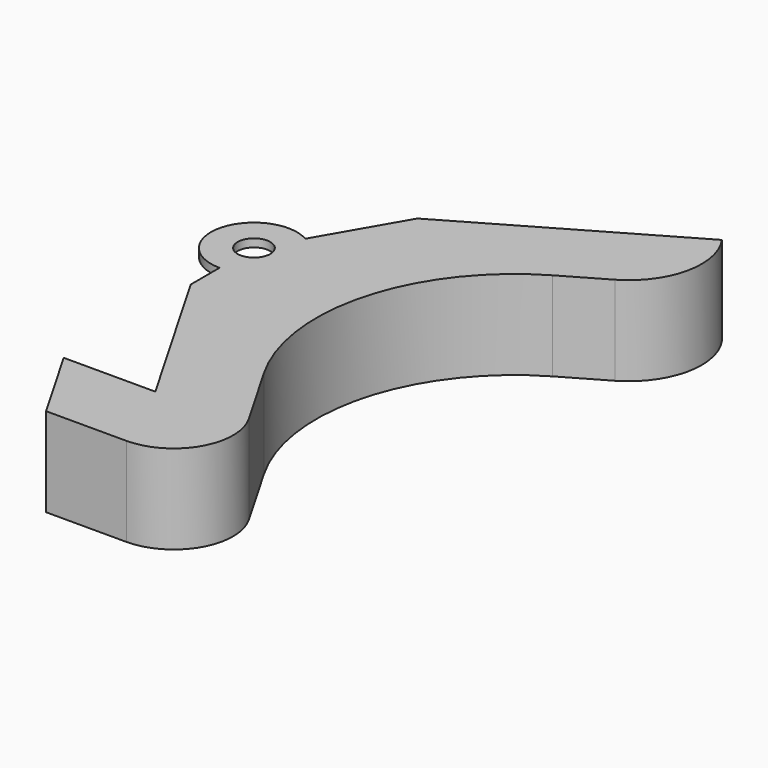
from build123d import *

# Parameters (mm, degrees)
F1_DEPTH    = 9
F2_T        = -1.625
F3_R        = 4.65
F4_DEPTH    = 5.75
F6_DEPTH    = 9
F7_T4_DEPTH = 11.5292765407
F8_R        = 1.5
F9_R        = 1.5
F11_DEPTH   = 25
F12_R       = 1.65
F13_DEPTH   = 0.8125
F14_R       = 4.65
F14_R_2     = 1.65
F15_DEPTH   = 0.8125
F17_DEPTH   = 25
F19_DEPTH   = 25


# Not quite as in the source:
# - a fillet or chamfer that OpenCascade refuses, or shapes differently, is made with other operations: its cross-section is extruded or revolved along the edge and cut away or added


with BuildPart() as f1:
    # F0 (on Top) → F1 (new body)
    with BuildSketch(Plane.XY):
        with BuildLine():
            Line((-2.2380131875, 10.0346875), (0, 9.35))
            Line((0, 9.35), (9.2696152423, -6.7054445662))
            Line((9.2696152423, -6.7054445662), (0, -6.7054445662))
            Line((0, -6.7054445662), (4.6188021535, -14.7054445662))
            Line((4.6188021535, -14.7054445662), (12.7337168574, -14.7054445662))
            ThreePointArc((12.7337168574, -14.7054445662), (17.9298692801, -11.7054445662), (17.9298692801, -5.7054445662))
            Line((17.9298692801, -5.7054445662), (14, 1.101288694))
            ThreePointArc((14, 1.101288694), (12.0019915499, 16.2776695961), (21.3205080757, 28.4217967697))
            Line((21.3205080757, 28.4217967697), (25.6506350946, 30.9217967697))
            ThreePointArc((25.6506350946, 30.9217967697), (29.1558482852, 35.7019755006), (28, 41.5158075373))
            Line((28, 41.5158075373), (-6.2733497352, 21.7280798417))
            ThreePointArc((-6.2733497352, 21.7280798417), (-7.2315061235, 14.8544401058), (-2.2380131875, 10.0346875))
        make_face()
        with BuildLine():
            ThreePointArc((1.65, 17.35), (1.166726189, 16.183273811), (0, 15.7))
            ThreePointArc((0, 15.7), (-1.166726189, 18.516726189), (1.65, 17.35))
        make_face(mode=Mode.SUBTRACT)
    extrude(amount=F1_DEPTH)

    # F2
    f2_openings = [f1.faces().sort_by_distance(p)[0] for p in [
        (10.863325, 31.621944, 4.5),
        (-7.231506, 14.85444, 4.5),
        (4.634808, 1.322278, 4.5),
        (4.634808, -6.705445, 4.5),
        (2.309401, -10.705445, 4.5),
        (-1.119007, 9.692344, 4.5),
    ]]
    offset(amount=F2_T, openings=f2_openings)

    # F3 (on face) → F4 (cut, through all)
    with BuildSketch(Plane.XY.offset(1.625)):
        with Locations((0, 17.35)):
            Circle(F3_R)
    extrude(amount=F4_DEPTH, mode=Mode.SUBTRACT)

    # F5 (on face) → F6 (join)
    with BuildSketch(Plane.XY):
        Polygon((0, -6.7054445662), (4.6188021535, -14.7054445662), (6.9282032303, -14.7054445662), (2.3094010768, -6.7054445662), align=None)
    extrude(amount=F6_DEPTH)

    # F7: fillet of radius 2 on 2 edges, made by hand


with BuildPart() as f7_tool2:
    # F7_s3 → F7_t4 (new body)
    with BuildSketch(Plane.XY.offset(-1.2646382703)):
        with BuildLine():
            ThreePointArc((5.4117350132, -12.0796445662), (6.1446642818, -12.8125738348), (7.1458642818, -13.0808445662))
            Line((7.1458642818, -13.0808445662), (7.1458642818, -13.2810845662))
            ThreePointArc((7.1458642818, -13.2810845662), (6.5679366623, -13.2806845662), (5.9900090428, -13.2806845662))
            Line((5.9900090428, -13.2806845662), (5.816596116, -13.1805645662))
            ThreePointArc((5.816596116, -13.1805645662), (5.5276323063, -12.6800645662), (5.2383220864, -12.1797645662))
            Line((5.2383220864, -12.1797645662), (5.4117350132, -12.0796445662))
        make_face()
    extrude(amount=F7_T4_DEPTH)

    split(bisect_by=Plane.XY.offset(9), keep=Keep.BOTTOM)

    split(bisect_by=Plane.XY, keep=Keep.TOP)


with BuildPart() as f1_1:
    add(f1.part)

    # F7_t1: union F7_tool2
    add(f7_tool2.part)

    # F8
    f8_edges = [f1_1.edges().sort_by_distance(p)[0] for p in [
        (14.557643, -3.114578, 7.375),
    ]]
    fillet(f8_edges, radius=F8_R)

    # F9
    f9_edges = [f1_1.edges().sort_by_distance(p)[0] for p in [
        (10.432362, 16.698251, 1.625),
        (3.870747, -9.409775, 1.625),
        (27.584345, 36.123263, 1.625),
        (22.673072, 31.079088, 1.625),
        (14.557643, -3.114578, 1.625),
        (16.522578, -10.892945, 1.625),
        (9.91978, -13.080445, 1.625),
        (6.144664, -12.812574, 1.625),
    ]]
    fillet(f9_edges, radius=F9_R)

    # F10 (on face) → F11 (cut)
    with BuildSketch(Plane(origin=(0, 0, 0), x_dir=(1, 0, 0), z_dir=(0, 0, -1))):
        with BuildLine():
            ThreePointArc((0, -22), (-4.65, -17.35), (0, -12.7))
            Line((0, -12.7), (0, -9.35))
            Line((0, -9.35), (-2.2380131875, -10.0346875))
            ThreePointArc((-2.2380131875, -10.0346875), (-7.2315061235, -14.8544401058), (-6.2733497352, -21.7280798417))
            Line((-6.2733497352, -21.7280798417), (0, -25.35))
            Line((0, -25.35), (0, -22))
        make_face()
    extrude(amount=-F11_DEPTH, mode=Mode.SUBTRACT)

    # F12 (on face) → F13 (cut)
    with BuildSketch(Plane(origin=(0, 0, 0), x_dir=(1, 0, 0), z_dir=(0, 0, -1))):
        with BuildLine():
            ThreePointArc((0, -22), (3.2880465325, -20.6380465325), (4.65, -17.35))
            ThreePointArc((4.65, -17.35), (3.2880465325, -14.0619534675), (0, -12.7))
            ThreePointArc((0, -12.7), (-4.65, -17.35), (0, -22))
        make_face()
        with Locations((0, -17.35)):
            Circle(F12_R, mode=Mode.SUBTRACT)
        with Locations((0, -17.35)):
            Circle(F12_R)
    extrude(amount=-F13_DEPTH, mode=Mode.SUBTRACT)

    # F14 (on face) → F15 (cut)
    with BuildSketch(Plane(origin=(0, 0, 7.375), x_dir=(1, 0, 0), z_dir=(0, 0, -1))):
        with Locations((0, -17.35)):
            Circle(F14_R)
        with Locations((0, -17.35)):
            Circle(F14_R_2, mode=Mode.SUBTRACT)
    extrude(amount=-F15_DEPTH, mode=Mode.SUBTRACT)

    # F16 (on face) → F17 (cut)
    with BuildSketch(Plane(origin=(0, 0, 0), x_dir=(1, 0, 0), z_dir=(0, 0, -1))):
        with BuildLine():
            Line((6.9282032303, -29.35), (2.325, -21.3770181276))
            ThreePointArc((2.325, -21.3770181276), (1.2035085597, -21.8415550922), (0, -22))
            Line((0, -22), (0, -25.35))
            Line((0, -25.35), (6.9282032303, -29.35))
        make_face()
    extrude(amount=-F17_DEPTH, mode=Mode.SUBTRACT)

    # F18 (on face) → F19 (cut)
    with BuildSketch(Plane.XY.offset(9)):
        with BuildLine():
            Line((2.175, 21.1172105065), (2.325, 21.3770181276))
            ThreePointArc((2.325, 21.3770181276), (-4.4915550922, 18.5535085597), (0, 12.7))
            Line((0, 12.7), (0, 13))
            ThreePointArc((0, 13), (-4.2017773444, 18.4758628462), (2.175, 21.1172105065))
        make_face()
    extrude(amount=-F19_DEPTH, mode=Mode.SUBTRACT)


solid = f1_1.part
